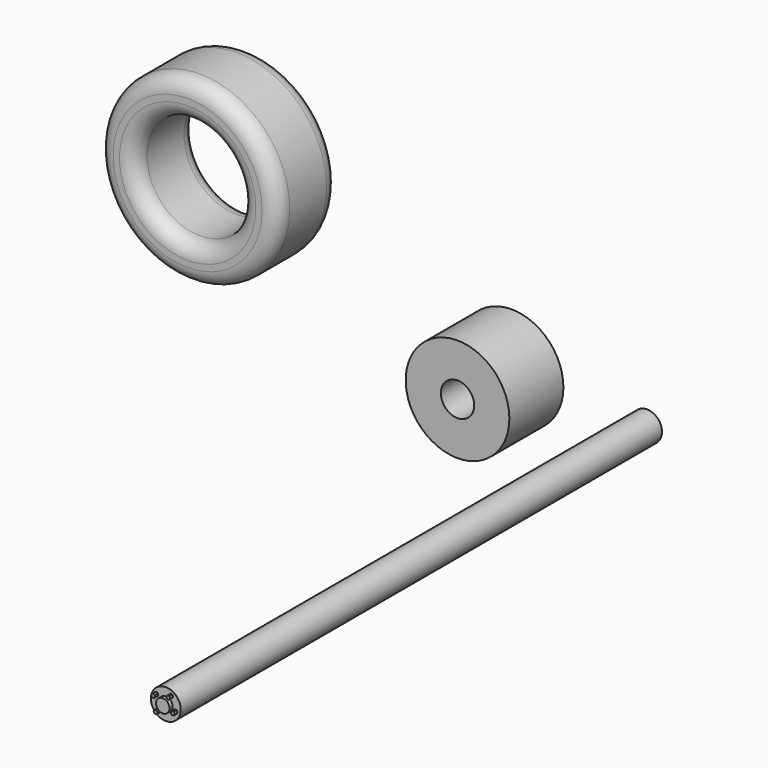
from build123d import *

# Parameters (mm, degrees)
F1_R      = 74.2769896622
F1_R_2    = 43.6656527846
F2_DEPTH  = 63.5
F3_R      = 12.7
F4_R      = 42.877056386
F4_R_2    = 13.7711488701
F5_DEPTH  = 55.88
F9_R      = 12.3612543208
F10_DEPTH = 497.6103901863
F11_R     = 5.5971792764
F12_DEPTH = 3.1027426012
F13_R     = 6.167140202
F14_DEPTH = 1.218579011


# Not quite as in the source:
# - the program builds the solid bodies; features that only make, move or delete a surface that nothing else refers to are left out


with BuildPart() as f2:
    # F1 (on face) → F2 (new body)
    with BuildSketch(Plane.XZ):
        Circle(F1_R)
        Circle(F1_R_2, mode=Mode.SUBTRACT)
    extrude(amount=F2_DEPTH)

    # F3
    f3_edges = [f2.edges().sort_by_distance(p)[0] for p in [
        (-74.27699, -63.5, 0),
        (-74.27699, 0, 0),
        (-43.665653, -63.5, 0),
        (-43.665653, 0, 0),
    ]]
    fillet(f3_edges, radius=F3_R)


with BuildPart() as f5:
    # F4 (on Front) → F5 (new body)
    with BuildSketch(Plane.XZ):
        with Locations((217.1535491943, -90.0512337685)):
            Circle(F4_R)
        with Locations((217.1535491943, -90.0512337685)):
            Circle(F4_R_2, mode=Mode.SUBTRACT)
    extrude(amount=F5_DEPTH)


with BuildPart() as f10:
    # F9 (on Front) → F10 (new body)
    with BuildSketch(Plane.XZ):
        with Locations((329.2273879051, -95.9801673889)):
            Circle(F9_R)
    extrude(amount=F10_DEPTH)

    # F11 (on face) → F12 (join)
    with BuildSketch(Plane.XZ.offset(497.6103901863)):
        Polygon((335.2533358502, -88.8653362571), (334.7347378731, -87.3432382941), (333.1572633815, -87.0313083352), (332.0983868671, -88.2414763392), (332.6169848442, -89.7635743022), (334.1944593358, -90.0755042611), align=None)
        Polygon((338.2459338014, -100.2556322923), (339.1215801239, -98.8398194313), (338.3332733805, -97.3735810408), (336.6693203146, -97.3231555113), (335.7936739922, -98.7389683723), (336.5819807356, -100.2052067628), align=None)
        Polygon((324.0882255018, -103.8427009407), (324.8517215252, -102.4203300476), (324.0016602098, -101.0479376491), (322.3881028711, -101.0979161438), (321.6246068478, -102.5202870369), (322.4746681631, -103.8926794354), align=None)
        Polygon((321.574677267, -92.9140994987), (322.9860663414, -91.9822081923), (322.8847193337, -90.2939637461), (321.3719832517, -89.5376106062), (319.9605941772, -90.4695019126), (320.0619411849, -92.1577463588), align=None)
        with Locations((329.2273879051, -95.9801673889)):
            Circle(F11_R)
    extrude(amount=F12_DEPTH)

    # F13 (on face) → F14 (join)
    with BuildSketch(Plane(origin=(0, 0, 0), x_dir=(-1, 0, 0), z_dir=(0, 1, 0))):
        with Locations((-329.2273879051, -95.9801673889)):
            Circle(F13_R)
        Polygon((-321.9546855155, -91.6545746838), (-320.5465078354, -91.2772491574), (-320.1691924867, -89.8690687502), (-321.2000548181, -88.8382138694), (-322.6082324982, -89.2155393958), (-322.9855478469, -90.623719803), align=None)
        Polygon((-338.0537469964, -92.3749109234), (-336.5919589996, -92.4425572157), (-335.8024815936, -91.2104348217), (-336.4747921844, -89.9106661354), (-337.9365801811, -89.8430198431), (-338.7260575871, -91.0751422371), align=None)
        Polygon((-335.1416822645, -103.525971147), (-334.3061506748, -102.2580638528), (-334.9864248065, -100.9005186234), (-336.5022305278, -100.8108806882), (-337.3377621174, -102.0787879825), (-336.6574879857, -103.4363332119), align=None)
        Polygon((-322.2323943953, -101.909467741), (-320.7257986069, -101.8995046616), (-319.9811289926, -100.5897728958), (-320.7430551667, -99.2900042095), (-322.2496509552, -99.299967289), (-322.9943205695, -100.6096990548), align=None)
    extrude(amount=F14_DEPTH)


solid = Compound([f2.part, f5.part, f10.part])
